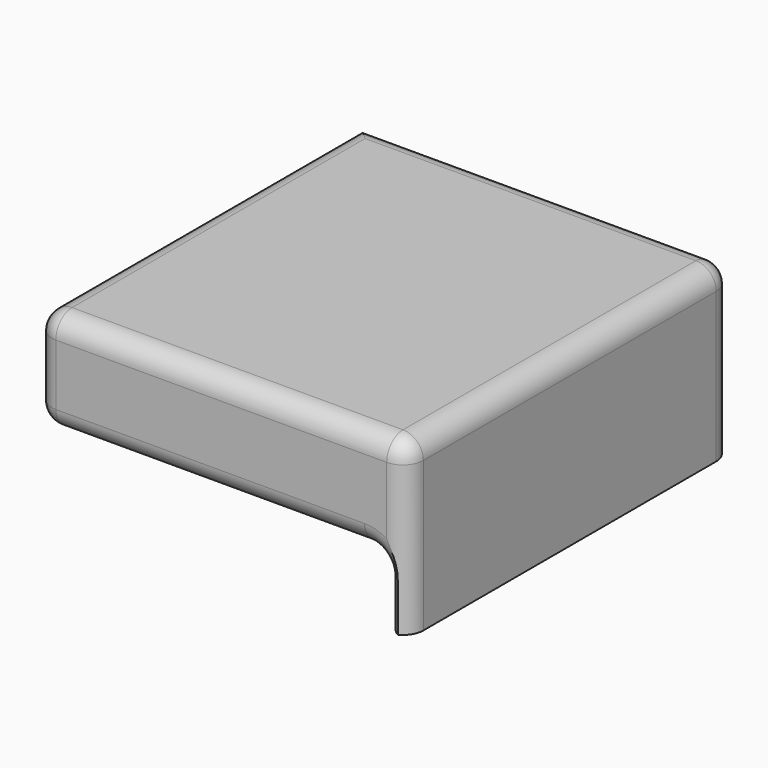
from build123d import *

# Parameters (mm, degrees)
F1_DEPTH     = 101.6
F2_T1_DEPTH  = 101.6
F2_T3_DEPTH  = 24.6862719756
F2_T5_DEPTH  = 127
F2_T7_DEPTH  = 94.8975325807
F2_T9_DEPTH  = 67.8662719756
F2_T11_DEPTH = 109.22
F2_T13_DEPTH = 100.4137670475
F2_T15_DEPTH = 50.0862719756
F2_S19_W     = 5.1816
F2_S19_H     = 5.1816
F2_T20_DEPTH = 5.1816
F2_T24_ANGLE = 90
F2_T26_ANGLE = 90
F3_T1_DEPTH  = 82.6337670475
F3_T3_DEPTH  = 15.24
F3_S7_W      = 5.08
F3_S7_H      = 5.08
F3_T8_DEPTH  = 5.08
F3_S13_W     = 5.08
F3_S13_H     = 5.08
F3_T14_DEPTH = 5.08
F3_T18_ANGLE = 89.9999999979


# Not quite as in the source:
# - a fillet or chamfer that OpenCascade refuses, or shapes differently, is made with other operations: its cross-section is extruded or revolved along the edge and cut away or added


with BuildPart() as f1:
    # F0 (on Front) → F1 (new body)
    with BuildSketch(Plane.XZ):
        Polygon((-47.2256254691, 25.4), (-128.5056254691, 25.4), (-128.5056254691, 0), (-41.2280928884, 0), (-41.2280928884, -17.0662719756), (-35.7118584216, -17.0662719756), (-35.7118584216, 25.4), align=None)
    extrude(amount=F1_DEPTH)

    # F2: fillet of radius 5.08 on 11 edges, made by hand

    # F2_s2 → F2_t1 (join)
    with BuildSketch(Plane.XZ):
        with BuildLine():
            ThreePointArc((-41.2280928884, -5.08), (-42.71599044, -1.4878975516), (-46.3080928884, 0))
            Line((-46.3080928884, 0), (-41.2280928884, 0))
            Line((-41.2280928884, 0), (-41.2280928884, -5.08))
        make_face()
    extrude(amount=F2_T1_DEPTH)

    # F2_s4 → F2_t3 (cut)
    with BuildSketch(Plane.XY.offset(-29.7662719756)):
        with BuildLine():
            ThreePointArc((-36.1480928884, 0), (-39.7401953368, -1.4878975516), (-41.2280928884, -5.08))
            Line((-41.2280928884, -5.08), (-41.2280928884, 0))
            Line((-41.2280928884, 0), (-36.1480928884, 0))
        make_face()
        with BuildLine():
            ThreePointArc((-36.1480928884, -101.6), (-39.7401953368, -100.1121024484), (-41.2280928884, -96.52))
            Line((-41.2280928884, -96.52), (-41.2280928884, -101.6))
            Line((-41.2280928884, -101.6), (-36.1480928884, -101.6))
        make_face()
    extrude(amount=F2_T3_DEPTH, mode=Mode.SUBTRACT)

    # F2_s6 → F2_t5 (cut)
    with BuildSketch(Plane.XZ.offset(-12.7)):
        with BuildLine():
            ThreePointArc((-128.5056254691, 5.08), (-127.0177279175, 1.4878975516), (-123.4256254691, 0))
            Line((-123.4256254691, 0), (-128.5056254691, 0))
            Line((-128.5056254691, 0), (-128.5056254691, 5.08))
        make_face()
        with BuildLine():
            ThreePointArc((-123.4256254691, 25.4), (-127.0177279175, 23.9121024484), (-128.5056254691, 20.32))
            Line((-128.5056254691, 20.32), (-128.5056254691, 25.4))
            Line((-128.5056254691, 25.4), (-123.4256254691, 25.4))
        make_face()
    extrude(amount=F2_T5_DEPTH, mode=Mode.SUBTRACT)

    # F2_s8 → F2_t7 (cut)
    with BuildSketch(Plane.YZ.offset(-141.2056254691)):
        with BuildLine():
            ThreePointArc((0, 5.08), (-1.4878975516, 1.4878975516), (-5.08, 0))
            Line((-5.08, 0), (0, 0))
            Line((0, 0), (0, 5.08))
        make_face()
        with BuildLine():
            ThreePointArc((-101.6, 5.08), (-100.1121024484, 1.4878975516), (-96.52, 0))
            Line((-96.52, 0), (-101.6, 0))
            Line((-101.6, 0), (-101.6, 5.08))
        make_face()
    extrude(amount=F2_T7_DEPTH, mode=Mode.SUBTRACT)

    # F2_s10 → F2_t9 (cut)
    with BuildSketch(Plane.XY.offset(-29.7662719756)):
        with BuildLine():
            ThreePointArc((-35.7118584216, -96.52), (-37.1997559731, -100.1121024484), (-40.7918584216, -101.6))
            Line((-40.7918584216, -101.6), (-35.7118584216, -101.6))
            Line((-35.7118584216, -101.6), (-35.7118584216, -96.52))
        make_face()
    extrude(amount=F2_T9_DEPTH, mode=Mode.SUBTRACT)

    # F2_s12 → F2_t11 (cut)
    with BuildSketch(Plane.XZ.offset(5.08)):
        with BuildLine():
            ThreePointArc((-40.7918584216, 25.4), (-37.1997559731, 23.9121024484), (-35.7118584216, 20.32))
            Line((-35.7118584216, 20.32), (-35.7118584216, 25.4))
            Line((-35.7118584216, 25.4), (-40.7918584216, 25.4))
        make_face()
    extrude(amount=F2_T11_DEPTH, mode=Mode.SUBTRACT)

    # F2_s14 → F2_t13 (cut)
    with BuildSketch(Plane.YZ.offset(-141.2056254691)):
        with BuildLine():
            ThreePointArc((-5.08, 25.4), (-1.4878975516, 23.9121024484), (0, 20.32))
            Line((0, 20.32), (0, 25.4))
            Line((0, 25.4), (-5.08, 25.4))
        make_face()
    extrude(amount=F2_T13_DEPTH, mode=Mode.SUBTRACT)

    # F2_s16 → F2_t15 (cut)
    with BuildSketch(Plane.XY.offset(-29.7662719756)):
        with BuildLine():
            ThreePointArc((-40.7918584216, 0), (-37.1997559731, -1.4878975516), (-35.7118584216, -5.08))
            Line((-35.7118584216, -5.08), (-35.7118584216, 0))
            Line((-35.7118584216, 0), (-40.7918584216, 0))
        make_face()
    extrude(amount=F2_T15_DEPTH, mode=Mode.SUBTRACT)


with BuildPart() as f2_tool18:
    # F2_s19 → F2_t20 (new body)
    with BuildSketch(Plane.XY.offset(20.32)):
        with Locations((-38.2010584216, -2.4892)):
            Rectangle(F2_S19_W, F2_S19_H)
    extrude(amount=F2_T20_DEPTH)

    # F2_s21 → F2_t22 (revolve, cut)
    with BuildSketch(Plane(origin=(-40.7918584216, -5.08, 20.32), x_dir=(-0.7071067812, -0.7071067812, 0), z_dir=(-0.7071067812, 0.7071067812, 0))):
        with BuildLine():
            ThreePointArc((0, -5.08), (5.08, 0), (0, 5.08))
            Line((0, 5.08), (0, -5.08))
        make_face()
    revolve(axis=Axis((-40.7918584216, -5.08, 20.32), (0, 0, 1)), mode=Mode.SUBTRACT)


with BuildPart() as f1_1:
    add(f1.part)

    # F2_t17: cut F2_tool18
    add(f2_tool18.part, mode=Mode.SUBTRACT)

    # F2_s23 → F2_t24 (revolve, cut)
    with BuildSketch(Plane.XY.offset(-5.08)):
        with BuildLine():
            ThreePointArc((-36.1480928884, -101.6), (-39.7401953368, -100.1121024484), (-41.2280928884, -96.52))
            Line((-41.2280928884, -96.52), (-41.2280928884, -101.6))
            Line((-41.2280928884, -101.6), (-36.1480928884, -101.6))
        make_face()
    revolve(axis=Axis((-46.3080928884, -101.6, -5.08), (0, -1, 0)), revolution_arc=F2_T24_ANGLE, mode=Mode.SUBTRACT)

    # F2_s25 → F2_t26 (revolve, cut)
    with BuildSketch(Plane.XY.offset(-5.08)):
        with BuildLine():
            ThreePointArc((-36.1480928884, 0), (-39.7401953368, -1.4878975516), (-41.2280928884, -5.08))
            Line((-41.2280928884, -5.08), (-41.2280928884, 0))
            Line((-41.2280928884, 0), (-36.1480928884, 0))
        make_face()
    revolve(axis=Axis((-46.3080928884, 0, -5.08), (0, -1, 0)), revolution_arc=F2_T26_ANGLE, mode=Mode.SUBTRACT)

    # F3: fillet of radius 5.08 on 3 edges, made by hand

    # F3_s2 → F3_t1 (cut)
    with BuildSketch(Plane.YZ.offset(-123.4256254691)):
        with BuildLine():
            ThreePointArc((-96.52, 25.4), (-100.1121024484, 23.9121024484), (-101.6, 20.32))
            Line((-101.6, 20.32), (-101.6, 25.4))
            Line((-101.6, 25.4), (-96.52, 25.4))
        make_face()
    extrude(amount=F3_T1_DEPTH, mode=Mode.SUBTRACT)

    # F3_s4 → F3_t3 (cut)
    with BuildSketch(Plane.XY.offset(5.08)):
        with BuildLine():
            ThreePointArc((-123.4256254691, -101.6), (-127.0177279175, -100.1121024484), (-128.5056254691, -96.52))
            Line((-128.5056254691, -96.52), (-128.5056254691, -101.6))
            Line((-128.5056254691, -101.6), (-123.4256254691, -101.6))
        make_face()
    extrude(amount=F3_T3_DEPTH, mode=Mode.SUBTRACT)


with BuildPart() as f3_tool6:
    # F3_s7 → F3_t8 (new body)
    with BuildSketch(Plane.XZ.offset(96.52)):
        with Locations((-125.9656254691, 2.54)):
            Rectangle(F3_S7_W, F3_S7_H)
    extrude(amount=F3_T8_DEPTH)

    # F3_s9 → F3_t10 (revolve, cut)
    with BuildSketch(Plane(origin=(-123.4256254691, -96.52, 5.08), x_dir=(0.7071067812, 0, 0.7071067812), z_dir=(0.7071067812, 0, -0.7071067812))):
        with BuildLine():
            ThreePointArc((0, -5.08), (5.08, 0), (0, 5.08))
            Line((0, 5.08), (0, -5.08))
        make_face()
    revolve(axis=Axis((-123.4256254691, -96.52, 5.08), (0, -1, 0)), mode=Mode.SUBTRACT)


with BuildPart() as f1_2:
    add(f1_1.part)

    # F3_t5: cut F3_tool6
    add(f3_tool6.part, mode=Mode.SUBTRACT)


with BuildPart() as f3_tool12:
    # F3_s13 → F3_t14 (new body)
    with BuildSketch(Plane.XY.offset(20.32)):
        with Locations((-38.2518584216, -99.06)):
            Rectangle(F3_S13_W, F3_S13_H)
    extrude(amount=F3_T14_DEPTH)

    # F3_s15 → F3_t16 (revolve, cut)
    with BuildSketch(Plane(origin=(-40.7918584216, -96.52, 20.32), x_dir=(-0.7071067812, 0.7071067812, 0), z_dir=(0.7071067812, 0.7071067812, 0))):
        with BuildLine():
            ThreePointArc((0, -5.08), (5.08, 0), (0, 5.08))
            Line((0, 5.08), (0, -5.08))
        make_face()
    revolve(axis=Axis((-40.7918584216, -96.52, 20.32), (0, 0, 1)), mode=Mode.SUBTRACT)


with BuildPart() as f1_3:
    add(f1_2.part)

    # F3_t11: cut F3_tool12
    add(f3_tool12.part, mode=Mode.SUBTRACT)

    # F3_s17 → F3_t18 (revolve, cut)
    with BuildSketch(Plane.XY.offset(20.3199999999)):
        with BuildLine():
            ThreePointArc((-128.5056254691, -96.52), (-127.0177279175, -100.1121024484), (-123.4256254691, -101.6))
            Line((-123.4256254691, -101.6), (-128.5056254691, -101.6))
            Line((-128.5056254691, -101.6), (-128.5056254691, -96.52))
        make_face()
    revolve(axis=Axis((-123.425625469, -101.6, 20.3199999999), (0, 1, 0)), revolution_arc=F3_T18_ANGLE, mode=Mode.SUBTRACT)


solid = f1_3.part
